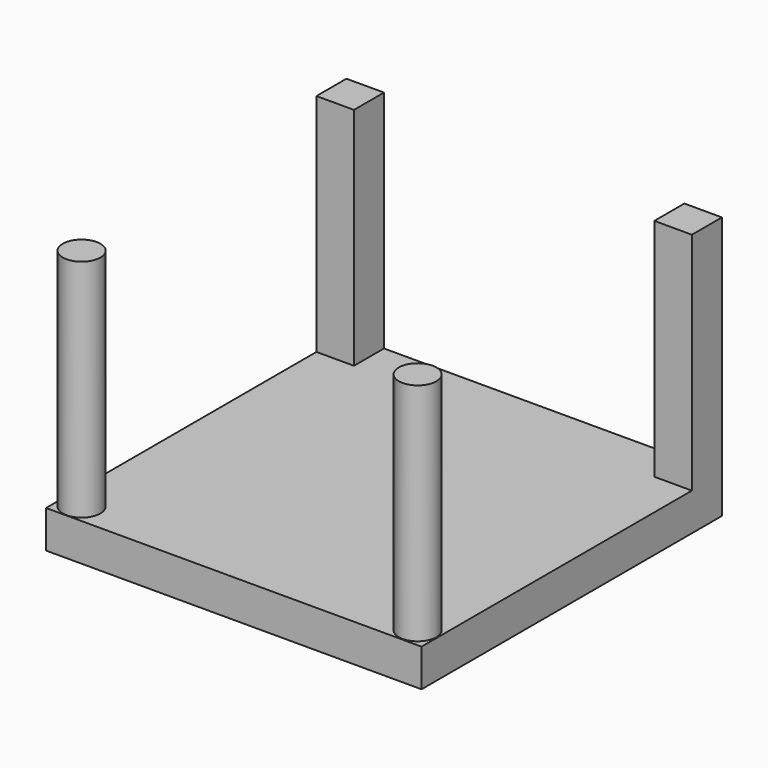
from build123d import *

# Parameters (mm, degrees)
F0_W     = 127
F0_H     = 127
F1_DEPTH = 12.7
F2_W     = 12.7
F2_H     = 12.7
F2_R     = 6.35
F3_DEPTH = 76.2


# Not quite as in the source:
# - a feature names something its author has since deleted; it is built from what else it names


with BuildPart() as f1:
    # F0 (on Top) → F1 (new body)
    with BuildSketch(Plane.XY):
        with Locations((-63.5, -63.5)):
            Rectangle(F0_W, F0_H)
    extrude(amount=F1_DEPTH)

    # F2 (on face) → F3 (join)
    with BuildSketch(Plane.XY.offset(12.7)):
        with Locations((-120.65, -6.35)):
            Rectangle(F2_W, F2_H)
        with Locations((-6.35, -6.35)):
            Rectangle(F2_W, F2_H)
        with Locations((-120.1874390244, -120.5023750663)):
            Circle(F2_R)
        with Locations((-6.6746613011, -120.3140169382)):
            Circle(F2_R)
    extrude(amount=F3_DEPTH)


solid = f1.part
